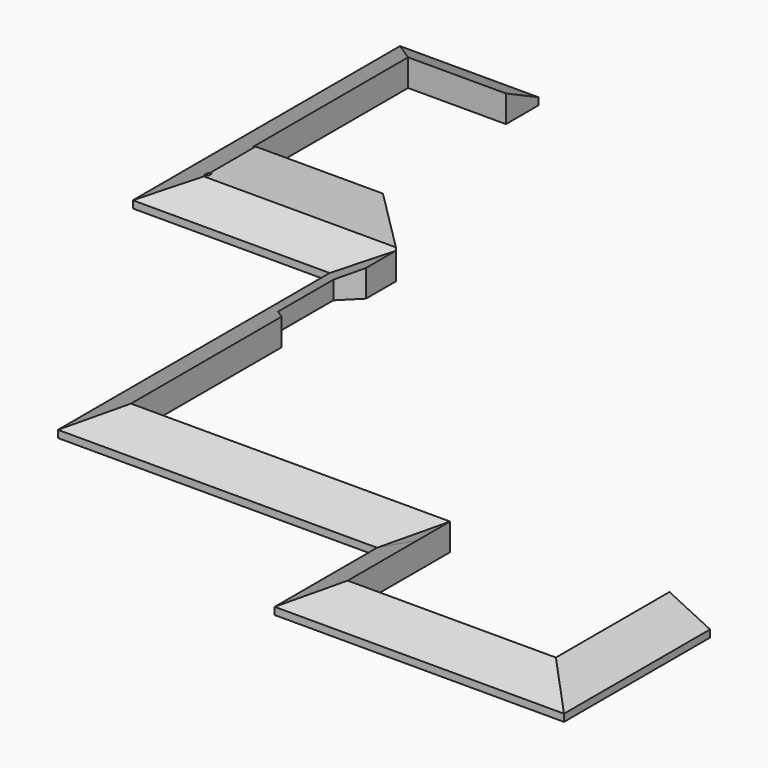
from build123d import *

# Parameters (mm, degrees)
F0_W        = 120
F0_H        = 120
F1_DEPTH    = 670
F2_T1_DEPTH = 3000
F2_T3_DEPTH = 4278.3373567146
F2_T5_DEPTH = 7960.6570053101
F2_T7_DEPTH = 7826.079643853
F3_T1_DEPTH = 10040.4964600443
F3_T3_DEPTH = 7529.4166998783
F3_T8_DEPTH = 12715.6483808339
F4_SIZE2    = 500
F4_SIZE     = 800


# Not quite as in the source:
# - a fillet or chamfer that OpenCascade refuses, or shapes differently, is made with other operations: its cross-section is extruded or revolved along the edge and cut away or added


with BuildPart() as f1:
    # F0 (on Top) → F1 (new body)
    with BuildSketch(Plane.XY):
        Polygon((-13984.2135623731, 12396.7366491631), (-17043.7082375624, 12396.7366491631), (-17043.7082375624, 16956.7366491631), (-14749.9399185181, 16956.7366491631), (-14749.9399185181, 17026.7366491631), (-14749.9399185181, 17906.7366491631), (-17993.7082375624, 17906.7366491631), (-17993.7082375624, 10080.6570053101), (-13380, 10080.6570053101), (-13380, 2120), (-5900, 2120), (-5900, -880), (880, -880), (880, 3398.3373567146), (-70, 3398.3373567146), (-70, 70), (-4950, 70), (-4950, 3070), (-12430, 3070), (-12430, 7483.9949493661), (-12854.2640687119, 7908.259018078), (-12854.2640687119, 9530.2691193458), (-12430, 9954.5331880577), (-12430, 10842.52308679), align=None)
        with Locations((-16983.7082375624, 11006.7366491631)):
            Rectangle(F0_W, F0_H, mode=Mode.SUBTRACT)
    extrude(amount=F1_DEPTH)

    # F2: chamfer of 500 x 1025.1519207896 on 4 edges, made by hand

    # F2_s2 → F2_t1 (cut)
    with BuildSketch(Plane.XZ.offset(-2120)):
        with BuildLine():
            Line((-5936.8560177183, 152.024119074), (-4837.992061492, 687.975880926))
            Line((-4837.992061492, 687.975880926), (-4837.992061492, 708.4789193418))
            ThreePointArc((-4837.992061492, 708.4789193418), (-5368.996030746, 690.5030384158), (-5900, 690.5030384158))
            Line((-5900, 690.5030384158), (-5920.5030384158, 670))
            ThreePointArc((-5920.5030384158, 670), (-5920.5030384158, 411.012059537), (-5957.3590561341, 152.024119074))
            Line((-5957.3590561341, 152.024119074), (-5936.8560177183, 152.024119074))
        make_face()
    extrude(amount=F2_T1_DEPTH, mode=Mode.SUBTRACT)

    # F2_s4 → F2_t3 (cut)
    with BuildSketch(Plane.XZ.offset(-3398.3373567146)):
        with BuildLine():
            Line((916.8560177183, 152.024119074), (-182.007938508, 687.975880926))
            Line((-182.007938508, 687.975880926), (-182.007938508, 708.4789193418))
            ThreePointArc((-182.007938508, 708.4789193418), (348.996030746, 690.5030384158), (880, 690.5030384158))
            Line((880, 690.5030384158), (900.5030384158, 670))
            ThreePointArc((900.5030384158, 670), (900.5030384158, 411.012059537), (937.3590561341, 152.024119074))
            Line((937.3590561341, 152.024119074), (916.8560177183, 152.024119074))
        make_face()
    extrude(amount=F2_T3_DEPTH, mode=Mode.SUBTRACT)

    # F2_s6 → F2_t5 (cut)
    with BuildSketch(Plane.XZ.offset(-10080.6570053101)):
        with BuildLine():
            Line((-13416.8560177183, 152.024119074), (-12317.992061492, 687.975880926))
            Line((-12317.992061492, 687.975880926), (-12317.992061492, 708.4789193418))
            ThreePointArc((-12317.992061492, 708.4789193418), (-12848.996030746, 690.5030384158), (-13380, 690.5030384158))
            Line((-13380, 690.5030384158), (-13400.5030384158, 670))
            ThreePointArc((-13400.5030384158, 670), (-13400.5030384158, 411.012059537), (-13437.3590561341, 152.024119074))
            Line((-13437.3590561341, 152.024119074), (-13416.8560177183, 152.024119074))
        make_face()
    extrude(amount=F2_T5_DEPTH, mode=Mode.SUBTRACT)

    # F2_s8 → F2_t7 (cut)
    with BuildSketch(Plane.XZ.offset(-17906.7366491631)):
        with BuildLine():
            Line((-18030.5642552807, 152.024119074), (-16931.7002990544, 687.975880926))
            Line((-16931.7002990544, 687.975880926), (-16931.7002990544, 708.4789193418))
            ThreePointArc((-16931.7002990544, 708.4789193418), (-17462.7042683084, 690.5030384158), (-17993.7082375624, 690.5030384158))
            Line((-17993.7082375624, 690.5030384158), (-18014.2112759782, 670))
            ThreePointArc((-18014.2112759782, 670), (-18014.2112759782, 411.012059537), (-18051.0672936965, 152.024119074))
            Line((-18051.0672936965, 152.024119074), (-18030.5642552807, 152.024119074))
        make_face()
    extrude(amount=F2_T7_DEPTH, mode=Mode.SUBTRACT)

    # F3: chamfer of 500 x 1025.1519207896 on 3 edges, made by hand

    # F3_s2 → F3_t1 (cut)
    with BuildSketch(Plane.YZ.offset(-7530.2482300221)):
        Polygon((-880, 170), (145.1519207896, 670), (-880, 670), align=None)
    extrude(amount=F3_T1_DEPTH, mode=Mode.SUBTRACT)

    # F3_s4 → F3_t3 (cut)
    with BuildSketch(Plane.YZ.offset(-19623.9564675845)):
        Polygon((17906.7366491631, 170), (16881.5847283734, 670), (17906.7366491631, 670), align=None)
    extrude(amount=F3_T3_DEPTH, mode=Mode.SUBTRACT)


with BuildPart() as f3_tool6:
    # F3_s7 → F3_t8 (new body)
    with BuildSketch(Plane.YZ.offset(-15010.2482300221)):
        Polygon((2120, 170), (3145.1519207896, 670), (2120, 670), align=None)
    extrude(amount=F3_T8_DEPTH)

    split(bisect_by=Plane(origin=(-1200.779561846, 0, 2461.9629485426), x_dir=(0, 1, 0), z_dir=(-0.4383711468, 0, 0.8987940463)), keep=Keep.TOP)


with BuildPart() as f1_1:
    add(f1.part)

    # F3_t5: cut F3_tool6
    add(f3_tool6.part, mode=Mode.SUBTRACT)

    # F4
    f4_edges = [f1_1.edges().sort_by_distance(p)[0] for p in [
        (-14699.278158, 10080.657005, 670),
    ]]
    f4_side = f1_1.faces().sort_by_distance((-14925.443793, 11155.7049, 670))[0]
    chamfer(f4_edges, length=F4_SIZE, length2=F4_SIZE2, reference=f4_side)


solid = f1_1.part
